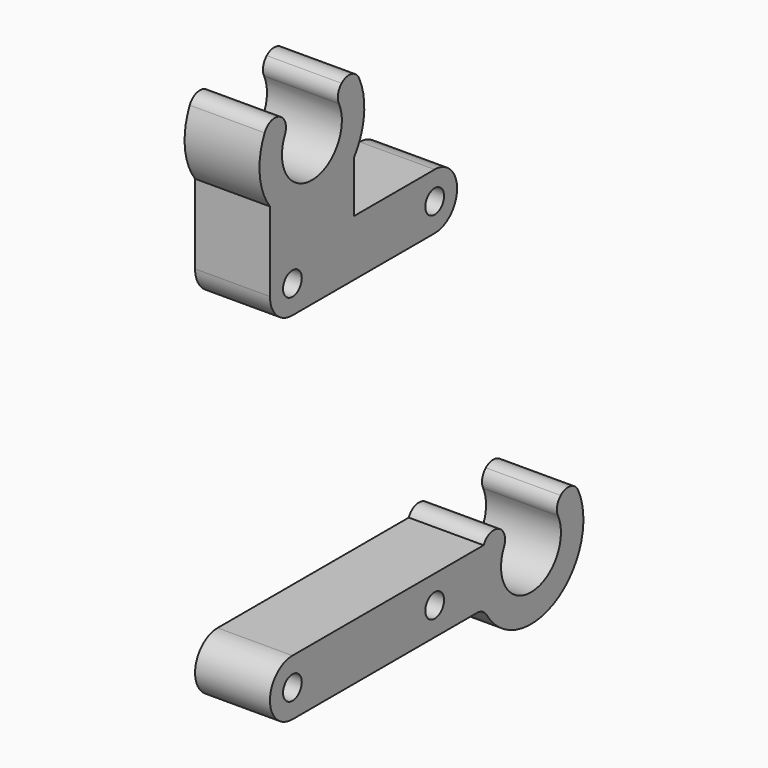
from build123d import *

# Parameters (mm, degrees)
F0_R     = 1.25
F1_DEPTH = 8
F2_R     = 1.49999
F3_R     = 1.49999


# Not quite as in the source:
# - a fillet or chamfer is up to 0.001 mm smaller than in the source, because OpenCascade refuses the exact size


with BuildPart() as f1:
    # F0 (on Right) → F1 (new body)
    with BuildSketch(Plane.YZ):
        with BuildLine():
            ThreePointArc((3, 53.3087513111), (0, 46.663), (-3, 53.3087513111))
            Line((-3, 53.3087513111), (-5.25, 55.2930647944))
            ThreePointArc((-5.25, 55.2930647944), (-6.9944413347, 50.9419093324), (-5.602, 46.4656679903))
            Line((-5.602, 46.4656679903), (-5.602, 38))
            ThreePointArc((-5.602, 38), (-4.7233203436, 35.8786796564), (-2.602, 35))
            Line((-2.602, 35), (16.398, 35))
            ThreePointArc((16.398, 35), (19.398, 38), (16.398, 41))
            Line((16.398, 41), (5.602, 41))
            Line((5.602, 41), (5.602, 46.4656679903))
            ThreePointArc((5.602, 46.4656679903), (6.9944413347, 50.9419093324), (5.25, 55.2930647944))
            Line((5.25, 55.2930647944), (3, 53.3087513111))
        make_face()
        with Locations((-2.602, 38)):
            Circle(F0_R, mode=Mode.SUBTRACT)
        with Locations((16.398, 38)):
            Circle(F0_R, mode=Mode.SUBTRACT)
    extrude(amount=F1_DEPTH)

    # F2 (radius 1.5 in the source; OpenCascade refuses exactly that, so slightly less here)
    f2_edges = [f1.edges().sort_by_distance(p)[0] for p in [
        (4, -5.25, 55.293065),
        (4, 5.25, 55.293065),
        (4, -3, 53.308751),
        (4, 3, 53.308751),
    ]]
    fillet(f2_edges, radius=F2_R)


with BuildPart() as f1b:
    # F0 (on Right) → F1, piece 2 (new body)
    with BuildSketch(Plane.YZ):
        with BuildLine():
            ThreePointArc((32.261, 2.6457513111), (29.261, -4), (26.261, 2.6457513111))
            Line((26.261, 2.6457513111), (24.011, 4.6300647944))
            ThreePointArc((24.011, 4.6300647944), (23.4166129043, 3.8526795189), (22.9364446797, 3))
            Line((22.9364446797, 3), (-2.602, 3))
            ThreePointArc((-2.602, 3), (-5.602, 0), (-2.602, -3))
            Line((-2.602, -3), (22.9364446797, -3))
            ThreePointArc((22.9364446797, -3), (33.1136795189, -5.8443870957), (34.511, 4.6300647944))
            Line((34.511, 4.6300647944), (32.261, 2.6457513111))
        make_face()
        with Locations((-2.602, 0)):
            Circle(F0_R, mode=Mode.SUBTRACT)
        with Locations((16.398, 0)):
            Circle(F0_R, mode=Mode.SUBTRACT)
    extrude(amount=F1_DEPTH)

    # F3 (radius 1.5 in the source; OpenCascade refuses exactly that, so slightly less here)
    f3_edges = [f1b.edges().sort_by_distance(p)[0] for p in [
        (4, 32.261, 2.645751),
        (4, 26.261, 2.645751),
        (4, 24.011, 4.630065),
        (4, 34.511, 4.630065),
        (4, 22.936445, -3),
    ]]
    fillet(f3_edges, radius=F3_R)


solid = Compound([f1.part, f1b.part])
